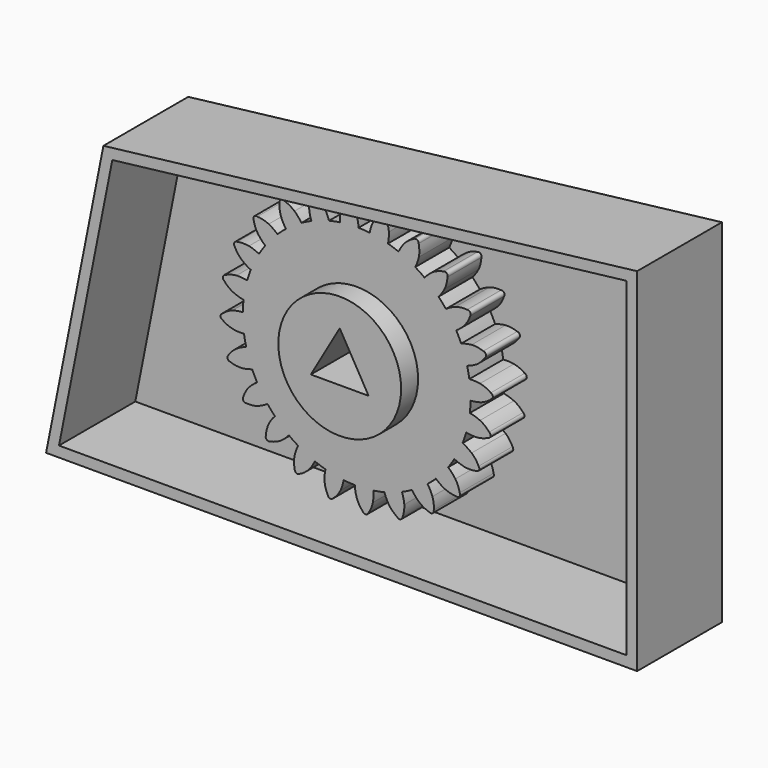
from build123d import *

# Parameters (mm, degrees)
F0_R     = 28.9693457265
F1_DEPTH = 25
F2_COUNT = 24
F3_DEPTH = 35
F5_DEPTH = 50
F6_T     = -5
F8_DEPTH = 30


with BuildPart() as f1:
    # F0 (on Front) → F1 (new body)
    with BuildSketch(Plane.XZ):
        with BuildLine():
            ThreePointArc((-7.8842675869, 53.139290225), (-35.0884247435, -40.6785974441), (53.721, 0))
            ThreePointArc((53.721, 0), (38.2966086664, 37.6738052983), (0.8807473744, 53.7137796572))
            ThreePointArc((0.8807473744, 53.7137796572), (-3.5135215054, 53.6059792153), (-7.8842675869, 53.139290225))
        make_face()
        Circle(F0_R, mode=Mode.SUBTRACT)
        with BuildLine():
            ThreePointArc((-7.8842675869, 53.139290225), (-3.5135215054, 53.6059792153), (0.8807473744, 53.7137796572))
            ThreePointArc((0.8807473744, 53.7137796572), (0.5961963294, 56.2215580315), (0, 58.674))
            ThreePointArc((0, 58.674), (-1.1998393393, 61.1918608506), (-2.8564405638, 63.4357213824))
            ThreePointArc((-2.8564405638, 63.4357213824), (-4.2093744174, 64.2226430613), (-5.448019844, 63.2658603022))
            ThreePointArc((-5.448019844, 63.2658603022), (-6.8256743808, 60.8371641198), (-7.6584938023, 58.1720357962))
            ThreePointArc((-7.6584938023, 58.1720357962), (-7.9294816777, 55.6627555721), (-7.8842675869, 53.139290225))
        make_face()
    extrude(amount=F1_DEPTH)


with BuildPart() as f2_1:
    # F2: instance of F1
    add(f1.part.rotate(Axis((0, 0, 0), (0, 1, 0)), 1 * 360 / F2_COUNT))


with BuildPart() as f2_2:
    # F2: instance of F1
    add(f1.part.rotate(Axis((0, 0, 0), (0, 1, 0)), 2 * 360 / F2_COUNT))


with BuildPart() as f2_3:
    # F2: instance of F1
    add(f1.part.rotate(Axis((0, 0, 0), (0, 1, 0)), 3 * 360 / F2_COUNT))


with BuildPart() as f2_4:
    # F2: instance of F1
    add(f1.part.rotate(Axis((0, 0, 0), (0, 1, 0)), 4 * 360 / F2_COUNT))


with BuildPart() as f2_5:
    # F2: instance of F1
    add(f1.part.rotate(Axis((0, 0, 0), (0, 1, 0)), 5 * 360 / F2_COUNT))


with BuildPart() as f2_6:
    # F2: instance of F1
    add(f1.part.rotate(Axis((0, 0, 0), (0, 1, 0)), 6 * 360 / F2_COUNT))


with BuildPart() as f2_7:
    # F2: instance of F1
    add(f1.part.rotate(Axis((0, 0, 0), (0, 1, 0)), 7 * 360 / F2_COUNT))


with BuildPart() as f2_8:
    # F2: instance of F1
    add(f1.part.rotate(Axis((0, 0, 0), (0, 1, 0)), 8 * 360 / F2_COUNT))


with BuildPart() as f2_9:
    # F2: instance of F1
    add(f1.part.rotate(Axis((0, 0, 0), (0, 1, 0)), 9 * 360 / F2_COUNT))


with BuildPart() as f2_10:
    # F2: instance of F1
    add(f1.part.rotate(Axis((0, 0, 0), (0, 1, 0)), 10 * 360 / F2_COUNT))


with BuildPart() as f2_11:
    # F2: instance of F1
    add(f1.part.rotate(Axis((0, 0, 0), (0, 1, 0)), 11 * 360 / F2_COUNT))


with BuildPart() as f2_12:
    # F2: instance of F1
    add(f1.part.rotate(Axis((0, 0, 0), (0, 1, 0)), 12 * 360 / F2_COUNT))


with BuildPart() as f2_13:
    # F2: instance of F1
    add(f1.part.rotate(Axis((0, 0, 0), (0, 1, 0)), 13 * 360 / F2_COUNT))


with BuildPart() as f2_14:
    # F2: instance of F1
    add(f1.part.rotate(Axis((0, 0, 0), (0, 1, 0)), 14 * 360 / F2_COUNT))


with BuildPart() as f2_15:
    # F2: instance of F1
    add(f1.part.rotate(Axis((0, 0, 0), (0, 1, 0)), 15 * 360 / F2_COUNT))


with BuildPart() as f2_16:
    # F2: instance of F1
    add(f1.part.rotate(Axis((0, 0, 0), (0, 1, 0)), 16 * 360 / F2_COUNT))


with BuildPart() as f2_17:
    # F2: instance of F1
    add(f1.part.rotate(Axis((0, 0, 0), (0, 1, 0)), 17 * 360 / F2_COUNT))


with BuildPart() as f2_18:
    # F2: instance of F1
    add(f1.part.rotate(Axis((0, 0, 0), (0, 1, 0)), 18 * 360 / F2_COUNT))


with BuildPart() as f2_19:
    # F2: instance of F1
    add(f1.part.rotate(Axis((0, 0, 0), (0, 1, 0)), 19 * 360 / F2_COUNT))


with BuildPart() as f2_20:
    # F2: instance of F1
    add(f1.part.rotate(Axis((0, 0, 0), (0, 1, 0)), 20 * 360 / F2_COUNT))


with BuildPart() as f2_21:
    # F2: instance of F1
    add(f1.part.rotate(Axis((0, 0, 0), (0, 1, 0)), 21 * 360 / F2_COUNT))


with BuildPart() as f2_22:
    # F2: instance of F1
    add(f1.part.rotate(Axis((0, 0, 0), (0, 1, 0)), 22 * 360 / F2_COUNT))


with BuildPart() as f2_23:
    # F2: instance of F1
    add(f1.part.rotate(Axis((0, 0, 0), (0, 1, 0)), 23 * 360 / F2_COUNT))


with BuildPart() as f1_1:
    add(f1.part)

    add(f2_1.part)  # F3 merges F2_1

    add(f2_2.part)  # F3 merges F2_2

    add(f2_3.part)  # F3 merges F2_3

    add(f2_4.part)  # F3 merges F2_4

    add(f2_5.part)  # F3 merges F2_5

    add(f2_6.part)  # F3 merges F2_6

    add(f2_7.part)  # F3 merges F2_7

    add(f2_8.part)  # F3 merges F2_8

    add(f2_9.part)  # F3 merges F2_9

    add(f2_10.part)  # F3 merges F2_10

    add(f2_11.part)  # F3 merges F2_11

    add(f2_12.part)  # F3 merges F2_12

    add(f2_13.part)  # F3 merges F2_13

    add(f2_14.part)  # F3 merges F2_14

    add(f2_15.part)  # F3 merges F2_15

    add(f2_16.part)  # F3 merges F2_16

    add(f2_17.part)  # F3 merges F2_17

    add(f2_18.part)  # F3 merges F2_18

    add(f2_19.part)  # F3 merges F2_19

    add(f2_20.part)  # F3 merges F2_20

    add(f2_21.part)  # F3 merges F2_21

    add(f2_22.part)  # F3 merges F2_22

    add(f2_23.part)  # F3 merges F2_23
    # F0 (on Front) → F3 (join)
    with BuildSketch(Plane.XZ):
        Circle(F0_R)
        Polygon((-13.6407520447, -7.875491865), (0, 15.75098373), (13.6407520447, -7.875491865), align=None, mode=Mode.SUBTRACT)
    extrude(amount=F3_DEPTH)


with BuildPart() as f5:
    # F4 (on Front) → F5 (new body)
    with BuildSketch(Plane.XZ):
        Polygon((152.2921919823, 95.0862392783), (-99.474273622, 65.2920305729), (-126.5230327845, -71.019500494), (152.2921919823, -71.019500494), align=None)
    extrude(amount=F5_DEPTH)

    # F6
    f6_openings = [f5.faces().sort_by_distance(p)[0] for p in [
        (24.121165, -50, 3.424742),
    ]]
    offset(amount=F6_T, openings=f6_openings)

    # F7 (on face) → F8 (cut)
    with BuildSketch(Plane.XZ.offset(5)):
        Polygon((37.8056822732, -4.3591911208), (24.1649302285, 19.2672844741), (10.5241781838, -4.3591911208), align=None)
    extrude(amount=-F8_DEPTH, mode=Mode.SUBTRACT)


solid = Compound([f1_1.part, f5.part])
